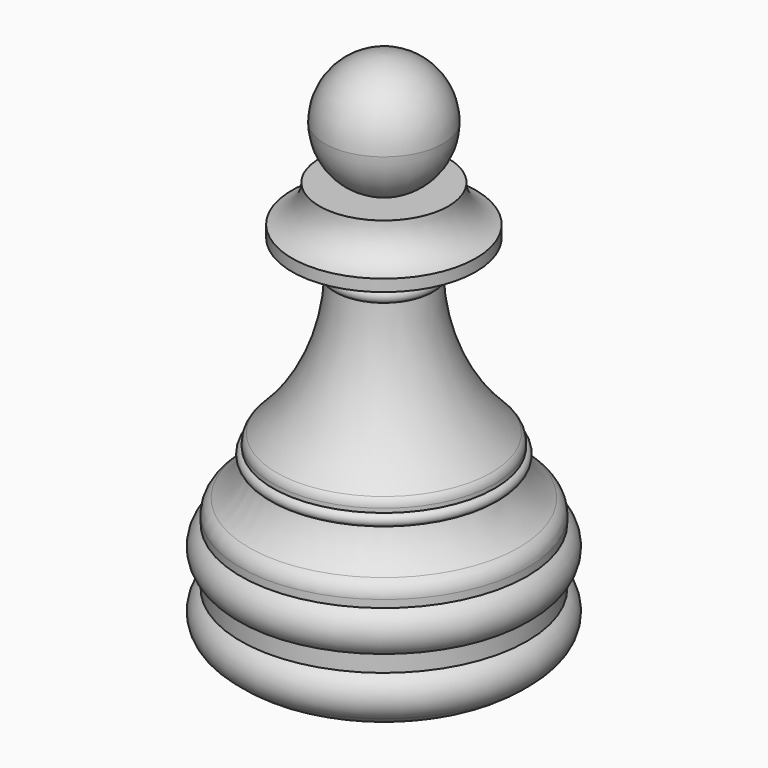
from build123d import *

# Parameters (mm, degrees)
F3_R        = 1.5
F5_R        = 1
F6_S5_R     = 9.379253336
F6_T6_DEPTH = 47009
F10_R       = 5
F11_DEPTH   = 10
F12_R       = 4.99999


# Not quite as in the source:
# - a fillet or chamfer that OpenCascade refuses, or shapes differently, is made with other operations: its cross-section is extruded or revolved along the edge and cut away or added
# - a fillet or chamfer is up to 0.001 mm smaller than in the source, because OpenCascade refuses the exact size


with BuildPart() as f1:
    # F0 (on Front) → F1 (revolve)
    with BuildSketch(Plane.XZ):
        with BuildLine():
            Line((-272.3507583141, 59.2592127276), (-277.7977287769, 59.2592127276))
            Line((-277.7977287769, 59.2592127276), (-277.7977287769, 24.2592127276))
            Line((-277.7977287769, 24.2592127276), (-265.6958699226, 24.2592127276))
            Line((-265.6958699226, 24.2592127276), (-265.6958699226, 25.6658904254))
            ThreePointArc((-265.6958699226, 25.6658904254), (-264.7929876455, 27.3731192574), (-265.6958699226, 29.0803480893))
            Line((-265.6958699226, 29.0803480893), (-265.6958699226, 30.4870257872))
            ThreePointArc((-265.6958699226, 30.4870257872), (-264.7929876455, 32.1942546192), (-265.6958699226, 33.9014834511))
            Line((-265.6958699226, 33.9014834511), (-265.6958699226, 36.0366143286))
            Line((-265.6958699226, 36.0366143286), (-268.4184754409, 36.0366143286))
            Line((-268.4184754409, 36.0366143286), (-268.4184754409, 38.5638475418))
            ThreePointArc((-268.4184754409, 38.5638475418), (-268.0457260693, 39.0616841614), (-268.4184754409, 39.559520781))
            Line((-268.4184754409, 39.559520781), (-268.4184754409, 40.9065671265))
            Line((-268.4184754409, 40.9065671265), (-273.8560736179, 40.9065671265))
            Line((-273.8560736179, 40.9065671265), (-273.8560736179, 52.3604340851))
            ThreePointArc((-273.8560736179, 52.3604340851), (-273.4234475816, 52.9374629259), (-273.8560736179, 53.5144917667))
            Line((-273.8560736179, 53.5144917667), (-273.8560736179, 55.1422908902))
            Line((-273.8560736179, 55.1422908902), (-270.0251638889, 55.1422908902))
            Line((-270.0251638889, 55.1422908902), (-270.0251638889, 56.1422908902))
            Line((-270.0251638889, 56.1422908902), (-272.3507583141, 56.1422908902))
            Line((-272.3507583141, 56.1422908902), (-272.3507583141, 59.2592127276))
        make_face()
    revolve(axis=Axis((-277.7977287769, 0, 41.7592127276), (0, 0, -1)))

    # F2: fillet of radius 5 on 1 edges, made by hand

    # F2_s1 → F2_t2 (revolve, cut)
    with BuildSketch(Plane.XZ):
        with BuildLine():
            ThreePointArc((-269.1726550516, 24.2592127276), (-267.2973699414, 24.6242040161), (-265.6958699226, 25.6658904254))
            Line((-265.6958699226, 25.6658904254), (-265.6958699226, 24.2592127276))
            Line((-265.6958699226, 24.2592127276), (-269.1726550516, 24.2592127276))
        make_face()
    revolve(axis=Axis((-277.7977287769, 0, 24.2592127276), (0, 0, -1)), mode=Mode.SUBTRACT)

    # F3
    f3_edges = [f1.edges().sort_by_distance(p)[0] for p in [
        (-289.899588, 0, 36.036614),
    ]]
    fillet(f3_edges, radius=F3_R)

    # F4: fillet of radius 5 on 1 edges, made by hand

    # F4_s1 → F4_t2 (revolve)
    with BuildSketch(Plane.XZ):
        with BuildLine():
            ThreePointArc((-266.3704491218, 35.7886050081), (-267.6414609661, 36.9939945683), (-268.4188594399, 38.5637355384))
            Line((-268.4188594399, 38.5637355384), (-268.8989893, 38.4236930284))
            ThreePointArc((-268.8989893, 38.4236930284), (-268.9186120094, 37.3001749335), (-268.9186120094, 36.0366143286))
            Line((-268.9186120094, 36.0366143286), (-268.4184754409, 35.5364777601))
            ThreePointArc((-268.4184754409, 35.5364777601), (-267.1958699226, 35.5364777601), (-266.6457379501, 35.3710494451))
            Line((-266.6457379501, 35.3710494451), (-266.3704491218, 35.7886050081))
        make_face()
    revolve(axis=Axis((-277.7977287769, 0, 36.0366143286), (0, 0, -1)))

    # F5
    f5_edges = [f1.edges().sort_by_distance(p)[0] for p in [
        (-287.176982, 0, 40.906567),
    ]]
    fillet(f5_edges, radius=F5_R)

    # F6: fillet of radius 17 on 1 edges, made by hand


with BuildPart() as f6_tool2:
    # F6_s3 → F6_t4 (revolve)
    with BuildSketch(Plane.XZ):
        with BuildLine():
            ThreePointArc((-268.7208850605, 40.6230639242), (-272.4364798651, 45.9894900588), (-273.8560736179, 52.3604340851))
            Line((-273.8560736179, 52.3604340851), (-275.5554961204, 52.3161265451))
            ThreePointArc((-275.5554961204, 52.3161265451), (-275.5560736179, 46.6335006058), (-275.5560736179, 40.9065671265))
            Line((-275.5560736179, 40.9065671265), (-273.8560736179, 39.2065671265))
            ThreePointArc((-273.8560736179, 39.2065671265), (-269.4184754409, 39.2065671265), (-269.9067887072, 39.4050193681))
            Line((-269.9067887072, 39.4050193681), (-268.7208850605, 40.6230639242))
        make_face()
    revolve(axis=Axis((-277.7977287769, 0, 40.9065671265), (0, 0, -1)))

    # F6_s5 → F6_t6 (intersect, symmetric)
    with BuildSketch(Plane.XY.offset(43.8)):
        with Locations((-277.7977287769, 0)):
            Circle(F6_S5_R)
    extrude(amount=F6_T6_DEPTH, both=True, mode=Mode.INTERSECT)


with BuildPart() as f1_1:
    add(f1.part)

    # F6_t1: union F6_tool2
    add(f6_tool2.part)

    # F7: fillet of radius 5.3 on 1 edges, made by hand

    # F7_s1 → F7_t2 (revolve)
    with BuildSketch(Plane.XZ):
        with BuildLine():
            ThreePointArc((-273.8560736179, 53.5144917667), (-272.111369605, 54.7183889535), (-270.0344325146, 55.1422908902))
            Line((-270.0344325146, 55.1422908902), (-273.8560736179, 55.1422908902))
            Line((-273.8560736179, 55.1422908902), (-273.8560736179, 53.5144917667))
        make_face()
    revolve(axis=Axis((-277.7977287769, 0, 55.1422908902), (0, 0, -1)))

    # F8: fillet of radius 3.25 on 1 edges, made by hand

    # F8_s1 → F8_t2 (revolve)
    with BuildSketch(Plane.XZ):
        with BuildLine():
            ThreePointArc((-270.0252777469, 56.141907437), (-271.705600505, 57.3142574044), (-272.3511583141, 59.2587738307))
            Line((-272.3511583141, 59.2587738307), (-272.6762948827, 59.2587738307))
            ThreePointArc((-272.6762948827, 59.2587738307), (-272.6758948827, 57.7005323605), (-272.6758948827, 56.1422908902))
            Line((-272.6758948827, 56.1422908902), (-272.3507583141, 55.8171543217))
            ThreePointArc((-272.3507583141, 55.8171543217), (-271.1880180305, 55.8171543217), (-270.1178262588, 55.8302207977))
            Line((-270.1178262588, 55.8302207977), (-270.0252777469, 56.141907437))
        make_face()
    revolve(axis=Axis((-277.7977287769, 0, 56.1422908902), (0, 0, -1)))


with BuildPart() as f11:
    # F10 (on offset) → F11 (new body)
    with BuildSketch(Plane.XY.offset(58.7592127276)):
        with Locations((-277.7977287769, 0)):
            Circle(F10_R)
    extrude(amount=F11_DEPTH)

    # F12 (radius 5 in the source; OpenCascade refuses exactly that, so slightly less here)
    f12_edges = [f11.edges().sort_by_distance(p)[0] for p in [
        (-282.797729, 0, 68.759213),
        (-282.797729, 0, 58.759213),
    ]]
    fillet(f12_edges, radius=F12_R)


solid = Compound([f1_1.part, f11.part])
